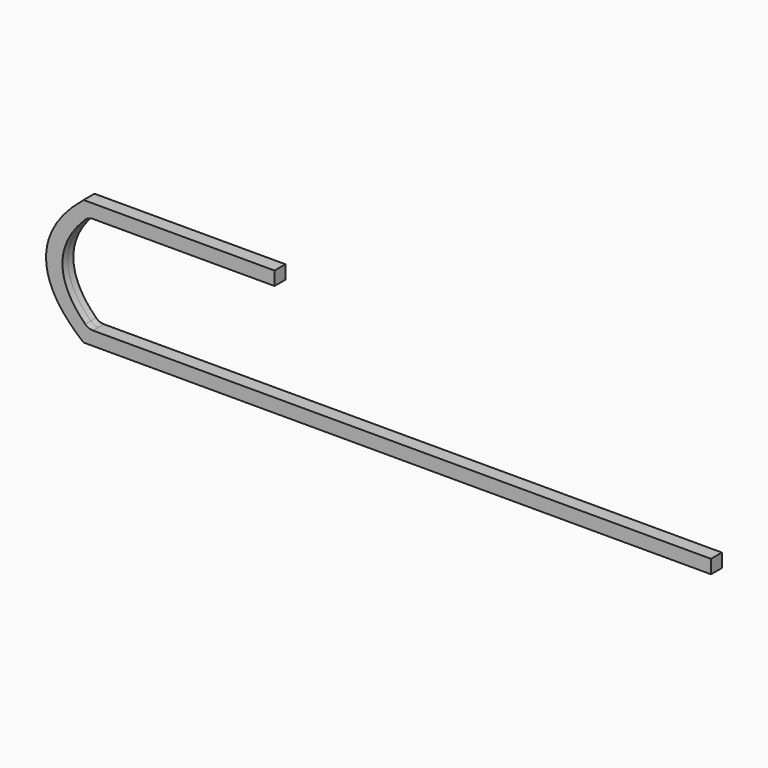
from build123d import *

# Parameters (mm, degrees)
F1_DEPTH = 12.5
F2_R     = 20


with BuildPart() as f1:
    # F0 (on Front) → F1 (new body, symmetric)
    with BuildSketch(Plane.XZ):
        with BuildLine():
            add(Edge.make_bspline(
                [(0, 230), (-143.18813182, 115), (0, 0)],
                knots=[5.8897826752, 5.8897826752, 5.8897826752, 6.6765879392, 6.6765879392, 6.6765879392], degree=2, weights=[1, 0.9236100668, 1]))
            Line((0, 0), (1150, 0))
            Line((1150, 0), (1150, 25))
            Line((1150, 25), (9.1600259417, 25))
            add(Edge.make_bspline(
                [(9.1600259417, 205), (-89.4541344002, 115), (9.1600259417, 25)],
                knots=[5.949769397, 5.949769397, 5.949769397, 6.6166012174, 6.6166012174, 6.6166012174], degree=2, weights=[1, 0.9449299244, 1]))
            Line((9.1600259417, 205), (350, 205))
            Line((350, 205), (350, 230))
            Line((350, 230), (0, 230))
        make_face()
    extrude(amount=F1_DEPTH, both=True)

    # F2
    f2_edges = [f1.edges().sort_by_distance(p)[0] for p in [
        (9.160026, -6.25, 25),
        (9.160026, 6.25, 25),
        (9.160026, -6.25, 205),
        (9.160026, 6.25, 205),
    ]]
    fillet(f2_edges, radius=F2_R)


solid = f1.part
